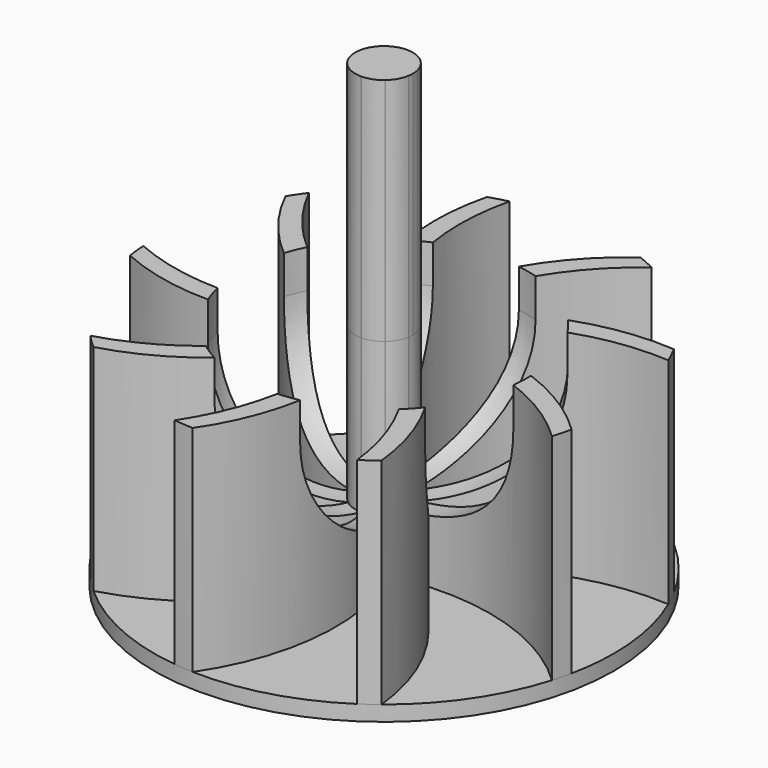
from build123d import *
from build123d import SkipClean  # not in build123d's __all__

# Parameters (mm, degrees)
F0_R     = 38.1
F1_DEPTH = 2.54
F3_DEPTH = 35.56
F7_DEPTH = 38.1
F8_R     = 3.2385
F9_DEPTH = 6.35


# Not quite as in the source:
# - after a boolean that leaves OpenCascade's solid faulty, fix() repairs it


with BuildPart() as f1:
    # F0 (on Top) → F1 (new body)
    with BuildSketch(Plane.XY):
        Circle(F0_R)
    extrude(amount=F1_DEPTH)

    # F2 (on face) → F3 (join)
    with BuildSketch(Plane.XY.offset(2.54)):
        with BuildLine():
            ThreePointArc((-25.4, -28.3980633142), (-9.8534313036, -19.639351751), (0, -4.7625))
            ThreePointArc((0, -4.7625), (0.0439522073, -4.7622971824), (0.0879006711, -4.7616887469))
            ThreePointArc((0.0879006711, -4.7616887469), (1.6759626521, -21.8194110942), (-4.3700858577, -37.8485448808))
            ThreePointArc((-4.3700858577, -37.8485448808), (-2.7892680291, -37.9977628797), (-1.2036056177, -38.0809838833))
            ThreePointArc((-1.2036056177, -38.0809838833), (5.075765672, -21.3782798302), (3.0612759911, -3.6482866604))
            ThreePointArc((3.0612759911, -3.6482866604), (3.0948149667, -3.6198793588), (3.1280903483, -3.5911637421))
            ThreePointArc((3.1280903483, -3.5911637421), (15.3091089785, -15.6373505938), (20.9808957068, -31.8027045287))
            ThreePointArc((20.9808957068, -31.8027045287), (22.2877879008, -30.9008820342), (23.5559692097, -29.9453888703))
            ThreePointArc((23.5559692097, -29.9453888703), (17.6299554789, -13.1140731837), (4.6901469237, -0.8269994461))
            ThreePointArc((4.6901469237, -0.8269994461), (4.6975794081, -0.7836797527), (4.7046117867, -0.7402933111))
            ThreePointArc((4.7046117867, -0.7402933111), (21.7789530721, -2.1383999607), (36.5146829934, -10.8760252799))
            ThreePointArc((36.5146829934, -10.8760252799), (36.9361401708, -9.3451350598), (37.2934442484, -7.798013599))
            ThreePointArc((37.2934442484, -7.798013599), (21.9348931821, 1.2863540521), (4.1244459855, 2.38125))
            ThreePointArc((4.1244459855, 2.38125), (4.1022942367, 2.4192123193), (4.0797930841, 2.4569685876))
            ThreePointArc((4.0797930841, 2.4569685876), (18.0581829771, 12.3611317796), (34.9628442919, 15.1396670709))
            ThreePointArc((34.9628442919, 15.1396670709), (34.3016619554, 16.5833044687), (33.5809022529, 17.9981389005))
            ThreePointArc((33.5809022529, 17.9981389005), (15.9762505862, 15.0848819308), (1.6288709326, 4.4752861065))
            ThreePointArc((1.6288709326, 4.4752861065), (1.5875, 4.4901280605), (1.5459938557, 4.504587578))
            ThreePointArc((1.5459938557, 4.504587578), (5.8877883728, 21.0767525816), (17.0515021775, 34.0713409406))
            ThreePointArc((17.0515021775, 34.0713409406), (15.6170548905, 34.7522315333), (14.1554828831, 35.3727621815))
            ThreePointArc((14.1554828831, 35.3727621815), (2.5421427847, 21.8250259042), (-1.6288709326, 4.4752861065))
            ThreePointArc((-1.6288709326, 4.4752861065), (-1.6701031298, 4.46006298), (-1.7111930797, 4.4444599778))
            ThreePointArc((-1.7111930797, 4.4444599778), (-9.0375678466, 19.9303266086), (-8.8384273121, 37.0606557234))
            ThreePointArc((-8.8384273121, 37.0606557234), (-10.3749457218, 36.6602032355), (-11.8934442484, 36.1960769132))
            ThreePointArc((-11.8934442484, 36.1960769132), (-12.0814618785, 18.3529976989), (-4.1244459855, 2.38125))
            ThreePointArc((-4.1244459855, 2.38125), (-4.146246444, 2.3430848631), (-4.1676937553, 2.3047201592))
            ThreePointArc((-4.1676937553, 2.3047201592), (-19.7341456292, 9.4582793146), (-30.5927584342, 22.7088778099))
            ThreePointArc((-30.5927584342, 22.7088778099), (-31.5123939262, 21.414458411), (-32.3772966351, 20.0828449827))
            ThreePointArc((-32.3772966351, 20.0828449827), (-21.0520162582, 6.2933978995), (-4.6901469237, -0.8269994461))
            ThreePointArc((-4.6901469237, -0.8269994461), (-4.6823149667, -0.8702487018), (-4.674084204, -0.9134238359))
            ThreePointArc((-4.674084204, -0.9134238359), (-21.1968973513, -5.4394019878), (-38.0323978843, -2.2686364119))
            ThreePointArc((-38.0323978843, -2.2686364119), (-37.9048427913, -3.8513494992), (-37.7114520927, -5.4273733112))
            ThreePointArc((-37.7114520927, -5.4273733112), (-20.1720982637, -8.7109527205), (-3.0612759911, -3.6482866604))
            ThreePointArc((-3.0612759911, -3.6482866604), (-3.0274762783, -3.6763832273), (-2.993418707, -3.7041666667))
            ThreePointArc((-2.993418707, -3.7041666667), (-12.7413852255, -17.7919266479), (-27.6762556813, -26.1846304435))
            ThreePointArc((-27.6762556813, -26.1846304435), (-26.561194449, -27.3150681757), (-25.4, -28.3980633142))
        make_face()
    extrude(amount=F3_DEPTH)

    # F4 (on Front) → F5 (revolve, cut)
    with BuildSketch(Plane.XZ):
        with BuildLine():
            Line((-4.7625, 12.7), (-4.7625, 44.45))
            Line((-4.7625, 44.45), (-23.8125, 44.45))
            Line((-23.8125, 44.45), (-23.8125, 31.75))
            ThreePointArc((-23.8125, 31.75), (-18.2328841816, 18.2796158184), (-4.7625, 12.7))
        make_face()
    with SkipClean():  # cleaning this boolean's faces spoils the solid; the shape is the same uncleaned
        revolve(axis=Axis((0, 0, 17.8491695515), (0, 0, 1)), mode=Mode.SUBTRACT)

    # F6 (on face) → F7 (join)
    with BuildSketch(Plane.XY.offset(38.1)):
        with BuildLine():
            ThreePointArc((4.7046117867, -0.7402933111), (4.7480058911, -0.3712765922), (4.7625, 0))
            ThreePointArc((4.7625, 0), (4.6002217477, 1.2326257023), (4.1244459855, 2.38125))
            ThreePointArc((4.1244459855, 2.38125), (4.1022942367, 2.4192123193), (4.0797930841, 2.4569685876))
            ThreePointArc((4.0797930841, 2.4569685876), (3.0274762783, 3.6763832273), (1.6288709326, 4.4752861065))
            ThreePointArc((1.6288709326, 4.4752861065), (1.5875, 4.4901280605), (1.5459938557, 4.504587578))
            ThreePointArc((1.5459938557, 4.504587578), (-0.0439522073, 4.7622971824), (-1.6288709326, 4.4752861065))
            ThreePointArc((-1.6288709326, 4.4752861065), (-1.6701031298, 4.46006298), (-1.7111930797, 4.4444599778))
            ThreePointArc((-1.7111930797, 4.4444599778), (-3.0948149667, 3.6198793588), (-4.1244459855, 2.38125))
            ThreePointArc((-4.1244459855, 2.38125), (-4.146246444, 2.3430848631), (-4.1676937553, 2.3047201592))
            ThreePointArc((-4.1676937553, 2.3047201592), (-4.6114015093, 1.1901186371), (-4.7625, 0))
            ThreePointArc((-4.7625, 0), (-4.7443772497, -0.4150792248), (-4.6901469237, -0.8269994461))
            ThreePointArc((-4.6901469237, -0.8269994461), (-4.6823149667, -0.8702487018), (-4.674084204, -0.9134238359))
            ThreePointArc((-4.674084204, -0.9134238359), (-4.1022942367, -2.4192123193), (-3.0612759911, -3.6482866604))
            ThreePointArc((-3.0612759911, -3.6482866604), (-3.0274762783, -3.6763832273), (-2.993418707, -3.7041666667))
            ThreePointArc((-2.993418707, -3.7041666667), (-1.5875, -4.4901280605), (0, -4.7625))
            ThreePointArc((0, -4.7625), (0.0439522073, -4.7622971824), (0.0879006711, -4.7616887469))
            ThreePointArc((0.0879006711, -4.7616887469), (1.6701031298, -4.46006298), (3.0612759911, -3.6482866604))
            ThreePointArc((3.0612759911, -3.6482866604), (3.0948149667, -3.6198793588), (3.1280903483, -3.5911637421))
            ThreePointArc((3.1280903483, -3.5911637421), (4.146246444, -2.3430848631), (4.6901469237, -0.8269994461))
            ThreePointArc((4.6901469237, -0.8269994461), (4.6975794081, -0.7836797527), (4.7046117867, -0.7402933111))
        make_face()
    extrude(amount=F7_DEPTH)

    add(f1.part.fix(), mode=Mode.REPLACE)

    # F8 (on face) → F9 (cut)
    with BuildSketch(Plane(origin=(0, 0, 0), x_dir=(1, 0, 0), z_dir=(0, 0, -1))):
        Circle(F8_R)
    extrude(amount=-F9_DEPTH, mode=Mode.SUBTRACT)


solid = f1.part
